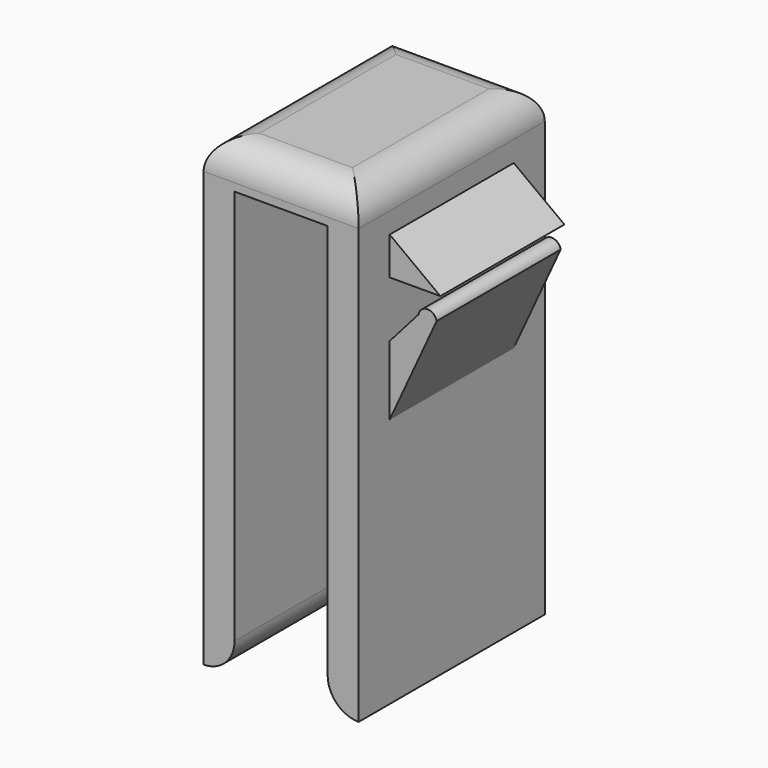
from build123d import *

# Parameters (mm, degrees)
F1_DEPTH = 19.05
F2_DEPTH = 12.7
F3_R     = 5.07999


# Not quite as in the source:
# - a fillet or chamfer is up to 0.001 mm smaller than in the source, because OpenCascade refuses the exact size


with BuildPart() as f1:
    # F0 (on Front) → F1 (new body, symmetric)
    with BuildSketch(Plane.XZ):
        Polygon((-8.1223546189, -57.6977613127), (-8.1223546189, 12.1522386873), (7.1176453811, 12.1522386873), (7.1176453811, -57.6977613127), (12.1976453811, -57.6977613127), (12.1976453811, -16.6773311794), (12.1976453811, -5.3586508704), (12.1976453811, 3.81), (12.1976453811, 9.9853777035), (12.1976453811, 18.5022386873), (-13.2023546189, 18.5022386873), (-13.2023546189, -57.6977613127), align=None)
    extrude(amount=F1_DEPTH, both=True)

    # F0 (on Front) → F2 (join, symmetric)
    with BuildSketch(Plane.XZ):
        Polygon((20.4923357815, 3.81), (12.1976453811, 9.9853777035), (12.1976453811, 3.81), (16.9246122241, 3.81), align=None)
        Polygon((12.1976453811, -5.3586508704), (12.1976453811, -16.6773311794), (19.8778546898, 0), (16.9246122241, 0), align=None)
        with BuildLine():
            Line((16.9246122241, 0), (19.8778546898, 0))
            ThreePointArc((19.8778546898, 0), (18.401233457, 1.2428820016), (16.9246122241, 0))
        make_face()
    extrude(amount=F2_DEPTH, both=True)

    # F3 (radius 5.08 in the source; OpenCascade refuses exactly that, so slightly less here)
    f3_edges = [f1.edges().sort_by_distance(p)[0] for p in [
        (12.197645, 0, 18.502239),
        (-13.202355, 0, 18.502239),
        (-0.502355, -19.05, 18.502239),
        (-0.502355, 19.05, 18.502239),
        (7.117645, 0, -57.697761),
        (-8.122355, 0, -57.697761),
    ]]
    fillet(f3_edges, radius=F3_R)


solid = f1.part
